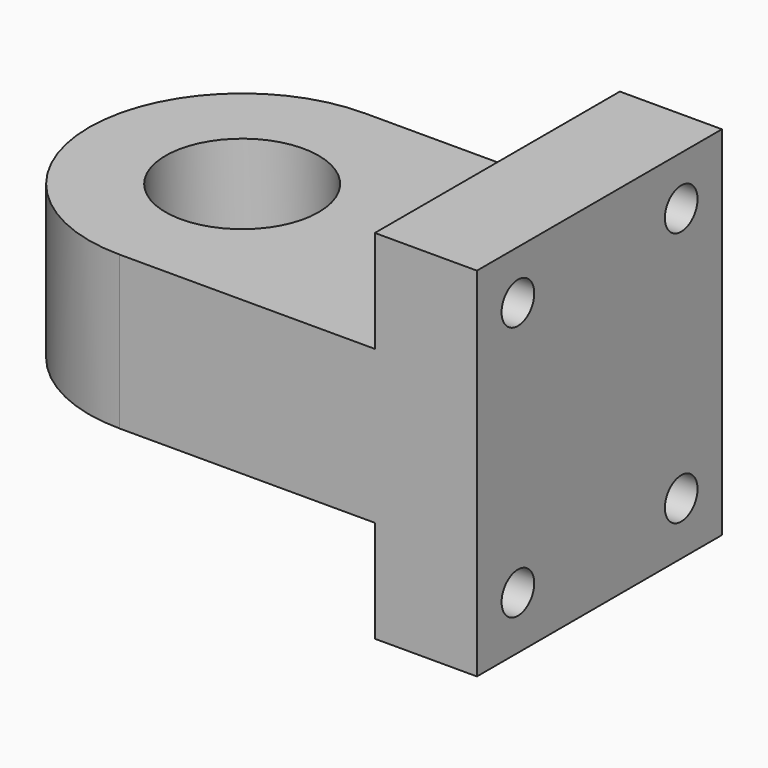
from build123d import *

# Parameters (mm, degrees)
F1_DEPTH = 30
F2_R     = 30
F3_R     = 29.99999
F4_R     = 15
F5_DEPTH = 15
F7_R     = 4
F8_DEPTH = 20


# Not quite as in the source:
# - a fillet or chamfer is up to 0.001 mm smaller than in the source, because OpenCascade refuses the exact size


with BuildPart() as f1:
    # F0 (on Front) → F1 (new body, symmetric)
    with BuildSketch(Plane.XZ):
        Polygon((-100, 0), (0, 0), (0, 35), (-20, 35), (-20, 15), (-100, 15), align=None)
    extrude(amount=F1_DEPTH, both=True)

    # F2
    f2_edges = [f1.edges().sort_by_distance(p)[0] for p in [
        (-100, -30, 7.5),
    ]]
    fillet(f2_edges, radius=F2_R)

    # F3 (radius 30 in the source; OpenCascade refuses exactly that, so slightly less here)
    f3_edges = [f1.edges().sort_by_distance(p)[0] for p in [
        (-100, 30, 7.5),
    ]]
    fillet(f3_edges, radius=F3_R)

    # F4 (on face) → F5 (cut, through all)
    with BuildSketch(Plane.XY.offset(15)):
        with Locations((-70, 0)):
            Circle(F4_R)
    extrude(amount=-F5_DEPTH, mode=Mode.SUBTRACT)

    # F6: F1 across plane


with BuildPart() as f1_1:
    add(f1.part)
    add(f1.part.mirror(Plane.XY))

    # F7 (on Right) → F8 (cut, through all)
    with BuildSketch(Plane.YZ):
        with Locations((-19.9676731229, 25.3771519661)):
            Circle(F7_R)
        with Locations((20.0323268771, 25.3771519661)):
            Circle(F7_R)
        with BuildLine():
            ThreePointArc((-23.9676731229, -24.6228480339), (-19.9676731229, -28.6228480339), (-15.9676731229, -24.6228480339))
            ThreePointArc((-15.9676731229, -24.6228480339), (-19.9676731229, -20.6228480339), (-23.9676731229, -24.6228480339))
        make_face()
        with Locations((20.0323268771, -24.6228480339)):
            Circle(F7_R)
    extrude(amount=-F8_DEPTH, mode=Mode.SUBTRACT)


solid = f1_1.part
